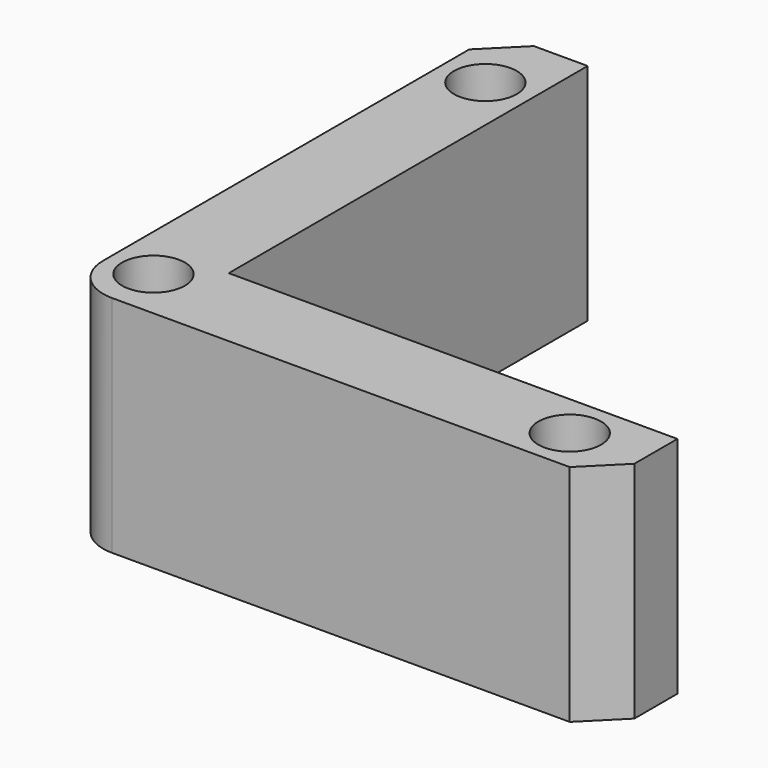
from build123d import *

# Parameters (mm, degrees)
F0_W        = 60
F0_H        = 60
F1_DEPTH    = 25
F2_W        = 50
F2_H        = 50
F3_DEPTH    = 25
F4_R        = 5
F5_R        = 2
F6_DEPTH    = 28
F7_R        = 3.5
F8_DEPTH    = 5
F9_S5_R     = 3.5
F9_T6_DEPTH = 12
F10_SIZE    = 4


# Not quite as in the source:
# - a fillet or chamfer that OpenCascade refuses, or shapes differently, is made with other operations: its cross-section is extruded or revolved along the edge and cut away or added


with BuildPart() as f1:
    # F0 (on Top) → F1 (new body)
    with BuildSketch(Plane.XY):
        with Locations((3.075433895, 2.043666031)):
            Rectangle(F0_W, F0_H)
    extrude(amount=F1_DEPTH)

    # F2 (on face) → F3 (cut)
    with BuildSketch(Plane.XY.offset(25)):
        with Locations((8.075433895, 7.043666031)):
            Rectangle(F2_W, F2_H)
    extrude(amount=-F3_DEPTH, mode=Mode.SUBTRACT)

    # F4
    f4_edges = [f1.edges().sort_by_distance(p)[0] for p in [
        (-26.924566, -27.956334, 12.5),
    ]]
    fillet(f4_edges, radius=F4_R)

    # F5 (on face) → F6 (cut)
    with BuildSketch(Plane.XY.offset(25)):
        with Locations((-21.924566105, 24.043666031)):
            Circle(F5_R)
        with Locations((-21.924566105, -22.1858429265)):
            Circle(F5_R)
        with Locations((25.075433895, -22.956333969)):
            Circle(F5_R)
    extrude(amount=-F6_DEPTH, mode=Mode.SUBTRACT)

    # F7 (on face) → F8 (cut)
    with BuildSketch(Plane.XY.offset(25)):
        with Locations((-21.924566105, 24.043666031)):
            Circle(F7_R)
        with Locations((25.075433895, -22.956333969)):
            Circle(F7_R)
        with Locations((-21.924566105, -22.1858429265)):
            Circle(F7_R)
    extrude(amount=-F8_DEPTH, mode=Mode.SUBTRACT)

    # F9: chamfer of 5 on 1 edges, made by hand


with BuildPart() as f9_tool2:
    # F9_s3 → F9_t4 (revolve)
    with BuildSketch(Plane.XZ.offset(22.1858429265)):
        Polygon((-19.924566105, 15), (-14.924566105, 20), (-19.924566105, 20), align=None)
    revolve(axis=Axis((-21.924566105, -22.1858429265, 20), (0, 0, 1)))

    # F9_s5 → F9_t6 (intersect, symmetric)
    with BuildSketch(Plane.XY.offset(17.5)):
        with Locations((-21.924566105, -22.1858429265)):
            Circle(F9_S5_R)
    extrude(amount=F9_T6_DEPTH, both=True, mode=Mode.INTERSECT)


with BuildPart() as f1_1:
    add(f1.part)

    # F9_t1: cut F9_tool2
    add(f9_tool2.part, mode=Mode.SUBTRACT)

    # F10
    f10_edges = [f1_1.edges().sort_by_distance(p)[0] for p in [
        (-26.924566, 32.043666, 12.5),
        (33.075434, -27.956334, 12.5),
    ]]
    chamfer(f10_edges, length=F10_SIZE)


solid = f1_1.part
